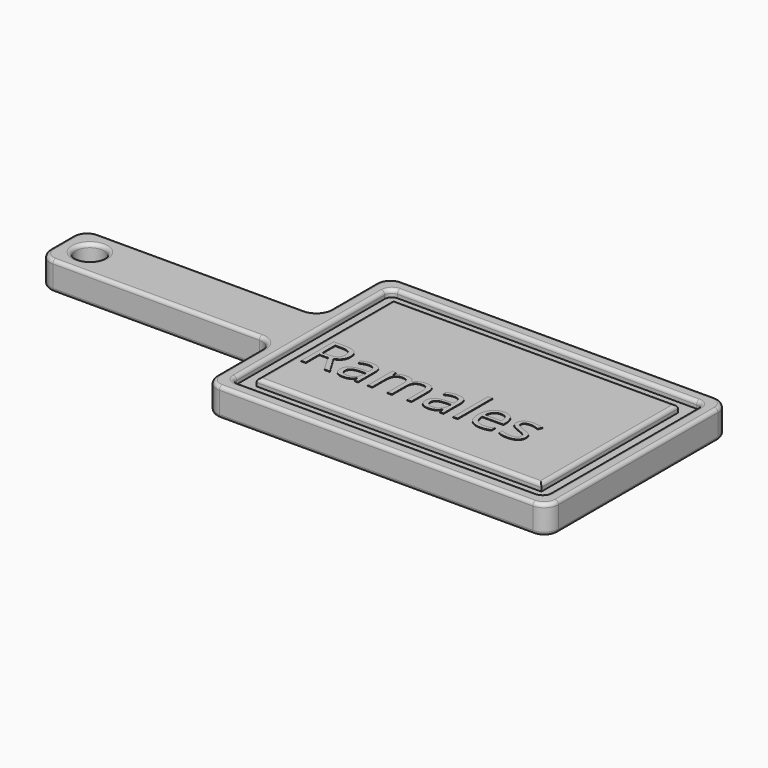
from build123d import *

# Parameters (mm, degrees)
F1_DEPTH     = 25.4
F2_R         = 12.7
F3_DEPTH     = 25.4
F5_DEPTH     = 6.35
F6_R         = 6.35
F7_R         = 12.7
F8_R         = 3.175
F9_TEXT_SIZE = 51.1778363701
F10_DEPTH    = 0.508


# Not quite as in the source:
# - Text() gives the source's letters only with a copy of the font that has no kerning and outlines rounded to 1/6400 em; it was checked with that copy


with BuildPart() as f1:
    # F0 (on Top) → F1 (new body)
    with BuildSketch(Plane.XY):
        Polygon((0, 76.2), (0, 0), (304.8, 0), (304.8, 203.2), (0, 203.2), (0, 127), (-209.5451450283, 127), (-209.5451450283, 76.2), align=None)
    extrude(amount=F1_DEPTH)

    # F2 (on face) → F3 (cut)
    with BuildSketch(Plane.XY.offset(25.4)):
        with Locations((-184.1451450283, 101.6)):
            Circle(F2_R)
    extrude(amount=-F3_DEPTH, mode=Mode.SUBTRACT)

    # F4 (on face) → F5 (cut)
    with BuildSketch(Plane.XY.offset(25.4)):
        Polygon((12.6999939203, 76.2), (12.6999939203, 12.6999939203), (292.1000060797, 12.6999939203), (292.1000060797, 190.5000060797), (12.6999939203, 190.5000060797), (12.6999939203, 127), align=None)
        Polygon((25.4000002861, 76.2), (25.4000002861, 127), (25.4000002861, 177.7999997139), (279.3999997139, 177.7999997139), (279.3999997139, 25.4000002861), (25.4000002861, 25.4000002861), align=None, mode=Mode.SUBTRACT)
    extrude(amount=-F5_DEPTH, mode=Mode.SUBTRACT)

    # F6
    f6_edges = [f1.edges().sort_by_distance(p)[0] for p in [
        (12.699994, 190.500006, 22.225),
        (292.100006, 190.500006, 22.225),
        (292.100006, 12.699994, 22.225),
        (12.699994, 12.699994, 22.225),
    ]]
    fillet(f6_edges, radius=F6_R)

    # F7
    f7_edges = [f1.edges().sort_by_distance(p)[0] for p in [
        (0, 0, 12.7),
        (-209.545145, 76.2, 12.7),
        (0, 127, 12.7),
        (0, 76.2, 12.7),
        (-209.545145, 127, 12.7),
        (0, 203.2, 12.7),
        (304.8, 203.2, 12.7),
        (304.8, 0, 12.7),
    ]]
    fillet(f7_edges, radius=F7_R)

    # F8
    f8_edges = [f1.edges().sort_by_distance(p)[0] for p in [
        (152.4, 177.8, 25.4),
        (279.4, 101.6, 25.4),
        (152.4, 25.4, 25.4),
        (25.4, 101.6, 25.4),
        (0, 38.1, 25.4),
        (-3.719744, 72.480256, 25.4),
        (3.719744, 3.719744, 25.4),
        (-104.772573, 76.2, 25.4),
        (152.4, 0, 25.4),
        (-205.825401, 79.919744, 25.4),
        (301.080256, 3.719744, 25.4),
        (-209.545145, 101.6, 25.4),
        (304.8, 101.6, 25.4),
        (-205.825401, 123.280256, 25.4),
        (301.080256, 199.480256, 25.4),
        (-104.772573, 127, 25.4),
        (152.4, 203.2, 25.4),
        (-3.719744, 130.719744, 25.4),
        (3.719744, 199.480256, 25.4),
        (0, 165.1, 25.4),
        (152.4, 12.699994, 25.4),
        (14.559866, 14.559866, 25.4),
        (290.240134, 14.559866, 25.4),
        (12.699994, 101.6, 25.4),
        (292.100006, 101.6, 25.4),
        (14.559866, 188.640134, 25.4),
        (290.240134, 188.640134, 25.4),
        (152.4, 190.500006, 25.4),
        (-196.845145, 101.6, 25.4),
        (0, 38.1, 0),
        (-3.719744, 72.480256, 0),
        (3.719744, 3.719744, 0),
        (-104.772573, 76.2, 0),
        (152.4, 0, 0),
        (-205.825401, 79.919744, 0),
        (301.080256, 3.719744, 0),
        (-209.545145, 101.6, 0),
        (304.8, 101.6, 0),
        (-205.825401, 123.280256, 0),
        (301.080256, 199.480256, 0),
        (-104.772573, 127, 0),
        (152.4, 203.2, 0),
        (-3.719744, 130.719744, 0),
        (3.719744, 199.480256, 0),
        (0, 165.1, 0),
        (-196.845145, 101.6, 0),
    ]]
    fillet(f8_edges, radius=F8_R)

    # F9 (on face) → F10 (join)
    with BuildSketch(Plane.XY.offset(25.4)):
        with Locations((28.5750002861, 64.7519578135)):
            Text('Ramales', F9_TEXT_SIZE, font='Open Sans', text_align=(TextAlign.LEFT, TextAlign.BOTTOM))
    extrude(amount=F10_DEPTH)


solid = f1.part
